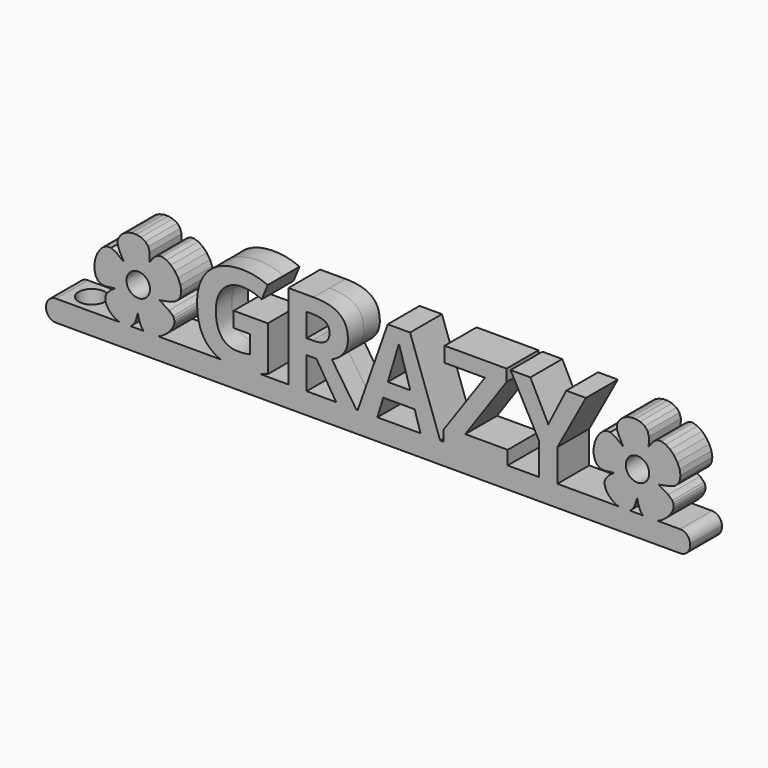
from build123d import *

# Parameters (mm, degrees)
F0_R         = 1.7660260944
F0_TEXT_SIZE = 18.1962925054
F1_DEPTH     = 3
F2_W         = 89.5
F2_H         = 6
F3_DEPTH     = 0.2
F4_DEPTH     = 3
F5_W         = 6
F5_H         = 3.2
F6_DEPTH     = 7.5
F7_R         = 1.5
F8_R         = 2
F9_DEPTH     = 4
F10_R        = 1.5


# Not quite as in the source:
# - Text() gives the source's letters only with a copy of the font that has no kerning and outlines rounded to 1/6400 em; it was checked with that copy


with BuildPart() as f1:
    # F0 (on Front) → F1 (new body, symmetric)
    with BuildSketch(Plane.XZ):
        Polygon((-9.8962181259, -0.0299609487), (-9.3093152472, 0.0995427735), (-8.5310452338, 0.4643787281), (-7.7886221935, 1.0156229815), (-7.1753136859, 1.6703047867), (-6.7844076966, 2.345448762), (-6.6844409889, 2.697736103), (-6.6652413988, 3.0240118702), (-6.7312263226, 3.3305926174), (-6.8868132072, 3.6238062576), (-7.4844896445, 4.1953846804), (-8.4936258745, 4.789299945), (-8.9274018823, 5.0567831788), (-8.4181052429, 5.1580766137), (-7.3131137554, 5.3695361907), (-6.5480905692, 5.6521941874), (-6.0523445823, 6.043851435), (-5.7552051187, 6.5823041299), (-5.6420905942, 7.3346827833), (-5.7751165223, 8.1369112107), (-6.1089634595, 8.9328581362), (-6.5983028952, 9.6663968681), (-7.1978267956, 10.281407439), (-7.8622157172, 10.7217585729), (-8.546147975, 10.9313258196), (-8.8812811082, 10.9320270148), (-9.2043064176, 10.8539824368), (-9.6469000392, 10.5612860557), (-10.1400767255, 9.9810366231), (-10.4508130024, 9.5801644376), (-10.4068223535, 10.0271686751), (-10.3916193646, 10.9311557532), (-10.598433195, 11.6324207168), (-11.0363252865, 12.1480644274), (-11.7143548393, 12.4951945719), (-12.3982545289, 12.6383143795), (-13.0712303381, 12.6247535348), (-13.7032208938, 12.4733707309), (-14.2641853, 12.2030313855), (-14.7240621838, 11.8325941916), (-15.0528129411, 11.3809291004), (-15.2203761991, 10.8668948051), (-15.1967042361, 10.3093544817), (-14.8286469794, 9.4077545862), (-14.3529716358, 8.5454741101), (-14.2906102139, 8.4004774316), (-14.4811582303, 8.5293860258), (-15.3946726039, 9.2300894295), (-16.21802192, 9.6332437342), (-16.8030362894, 9.634121823), (-17.3568401554, 9.3699870508), (-17.8525159958, 8.8932532172), (-18.2631576982, 8.2563454299), (-18.5618432066, 7.5116797807), (-18.7216618753, 6.7116836696), (-18.7156984739, 5.9087754295), (-18.5170445979, 5.1553756349), (-18.2008868091, 4.6439944488), (-17.7512302174, 4.3560670179), (-17.1086136552, 4.2712956407), (-16.2135760559, 4.3694053341), (-15.7044514474, 4.4302814773), (-15.6696932647, 4.4000047008), (-15.7790195709, 4.3290260096), (-16.1651405309, 4.0708069691), (-16.5523139664, 3.7127982689), (-16.8671052824, 3.3322639471), (-17.0360798838, 3.0064680418), (-17.0831036318, 2.6043628391), (-17.0239245605, 2.1921008316), (-16.867618816, 1.7819255621), (-16.6232807801, 1.3860941234), (-16.3000002503, 1.0168545414), (-15.9068693162, 0.6864593752), (-15.4529754831, 0.4071521172), (-14.9474063577, 0.1911989779), (-14.4397479673, 0.0570083052), (-13.9840845603, 0.0188926715), (-13.5797273957, 0.0772799851), (-13.2259605822, 0.2326232662), (-12.9220907946, 0.485341356), (-12.6674066752, 0.8358849825), (-12.4612081239, 1.2846821047), (-12.3027905578, 1.8321743328), (-12.1879723822, 2.2557758958), (-12.1309056827, 2.0998483864), (-12.0112204133, 1.5291342486), (-11.8237778137, 0.9902805659), (-11.5954117235, 0.5466869075), (-11.3529559319, 0.2617414835), (-10.9521058183, 0.053843468), (-10.4551700276, -0.0442881949), align=None)
        with Locations((-12.1185852993, 6.0541479067)):
            Circle(F0_R, mode=Mode.SUBTRACT)
        Polygon((65.0599232745, 9.9810366231), (64.7491869976, 9.5801644376), (64.7931776465, 10.0271686751), (64.8083806354, 10.9311557532), (64.601566805, 11.6324207168), (64.1636747135, 12.1480644274), (63.4856451607, 12.4951945719), (62.8017454711, 12.6383143795), (62.1287696619, 12.6247535348), (61.4967791062, 12.4733707309), (60.9358147, 12.2030313855), (60.4759378162, 11.8325941916), (60.1471870589, 11.3809291004), (59.9796238009, 10.8668948051), (60.0032957639, 10.3093544817), (60.3713530206, 9.4077545862), (60.8470283642, 8.5454741101), (60.9093897861, 8.4004774316), (60.7188417697, 8.5293860258), (59.8053273961, 9.2300894295), (58.98197808, 9.6332437342), (58.3969637106, 9.634121823), (57.8431598446, 9.3699870508), (57.3474840042, 8.8932532172), (56.9368423018, 8.2563454299), (56.6381567934, 7.5116797807), (56.4783381247, 6.7116836696), (56.4843015261, 5.9087754295), (56.6829554021, 5.1553756349), (56.9991131909, 4.6439944488), (57.4487697826, 4.3560670179), (58.0913863448, 4.2712956407), (58.9864239441, 4.3694053341), (59.4955485526, 4.4302814773), (59.5303067353, 4.4000047008), (59.4209804291, 4.3290260096), (59.0348594691, 4.0708069691), (58.6476860336, 3.7127982689), (58.3328947176, 3.3322639471), (58.1639201162, 3.0064680418), (58.1168963682, 2.6043628391), (58.1760754395, 2.1921008316), (58.332381184, 1.7819255621), (58.5767192199, 1.3860941234), (58.8999997497, 1.0168545414), (59.2931306838, 0.6864593752), (59.7470245169, 0.4071521172), (60.2525936423, 0.1911989779), (60.7602520327, 0.0570083052), (61.2159154397, 0.0188926715), (61.6202726043, 0.0772799851), (61.9740394178, 0.2326232662), (62.2779092054, 0.485341356), (62.5325933248, 0.8358849825), (62.7387918761, 1.2846821047), (62.8972094422, 1.8321743328), (63.0120276178, 2.2557758958), (63.0690943173, 2.0998483864), (63.1887795867, 1.5291342486), (63.3762221863, 0.9902805659), (63.6045882765, 0.5466869075), (63.8470440681, 0.2617414835), (64.2478941817, 0.053843468), (64.7448299724, -0.0442881949), (65.3037818741, -0.0299609487), (65.8906847528, 0.0995427735), (66.6689547662, 0.4643787281), (67.4113778065, 1.0156229815), (68.0246863141, 1.6703047867), (68.4155923034, 2.345448762), (68.5155590111, 2.697736103), (68.5347586012, 3.0240118702), (68.4687736774, 3.3305926174), (68.3131867928, 3.6238062576), (67.7155103555, 4.1953846804), (66.7063741255, 4.789299945), (66.2725981177, 5.0567831788), (66.7818947571, 5.1580766137), (67.8868862446, 5.3695361907), (68.6519094308, 5.6521941874), (69.1476554177, 6.043851435), (69.4447948813, 6.5823041299), (69.5579094058, 7.3346827833), (69.4248834777, 8.1369112107), (69.0910365405, 8.9328581362), (68.6016971048, 9.6663968681), (68.0021732044, 10.281407439), (67.3377842828, 10.7217585729), (66.653852025, 10.9313258196), (66.3187188918, 10.9320270148), (65.9956935824, 10.8539824368), (65.5530999608, 10.5612860557), align=None)
        with Locations((63.0814147007, 6.0541479067)):
            Circle(F0_R, mode=Mode.SUBTRACT)
        with Locations((-4.3154213579, 0)):
            Text('GRAZY', F0_TEXT_SIZE, font='Open Sans', font_style=FontStyle.BOLD, text_align=(TextAlign.LEFT, TextAlign.BOTTOM))
    extrude(amount=F1_DEPTH, both=True)



with BuildPart() as f3:
    # F2 (on Top) → F3 (new body)
    with BuildSketch(Plane.XY):
        with Locations((26.25, 0)):
            Rectangle(F2_W, F2_H)
    extrude(amount=F3_DEPTH)


with BuildPart() as f4:
    # F4 (new): a face of the model
    f4_faces = [f3.part.faces().sort_by_distance(p)[0] for p in [
        (26.25, 0, 0),
    ]]
    extrude(f4_faces, amount=F4_DEPTH)


with BuildPart() as f1_1:
    add(f1.part)

    add(f3.part)  # F6 merges F3

    add(f4.part)  # F6 merges F4
    # F5 (on face) → F6 (join)
    with BuildSketch(Plane(origin=(-18.5, 0, 0), x_dir=(0, -1, 0), z_dir=(-1, 0, 0))):
        with Locations((0, -1.4)):
            Rectangle(F5_W, F5_H)
    extrude(amount=F6_DEPTH)

    # F7
    f7_edges = [f1_1.edges().sort_by_distance(p)[0] for p in [
        (-26, 0, -3),
        (-26, 0, 0.2),
        (71, 0, -3),
    ]]
    fillet(f7_edges, radius=F7_R)

    # F8 (on face) → F9 (cut)
    with BuildSketch(Plane.XY.offset(0.2)):
        with Locations((-21.5, 0)):
            Circle(F8_R)
    extrude(amount=-F9_DEPTH, mode=Mode.SUBTRACT)

    # F10
    f10_edges = [f1_1.edges().sort_by_distance(p)[0] for p in [
        (71, 0, 0.2),
    ]]
    fillet(f10_edges, radius=F10_R)


solid = f1_1.part
